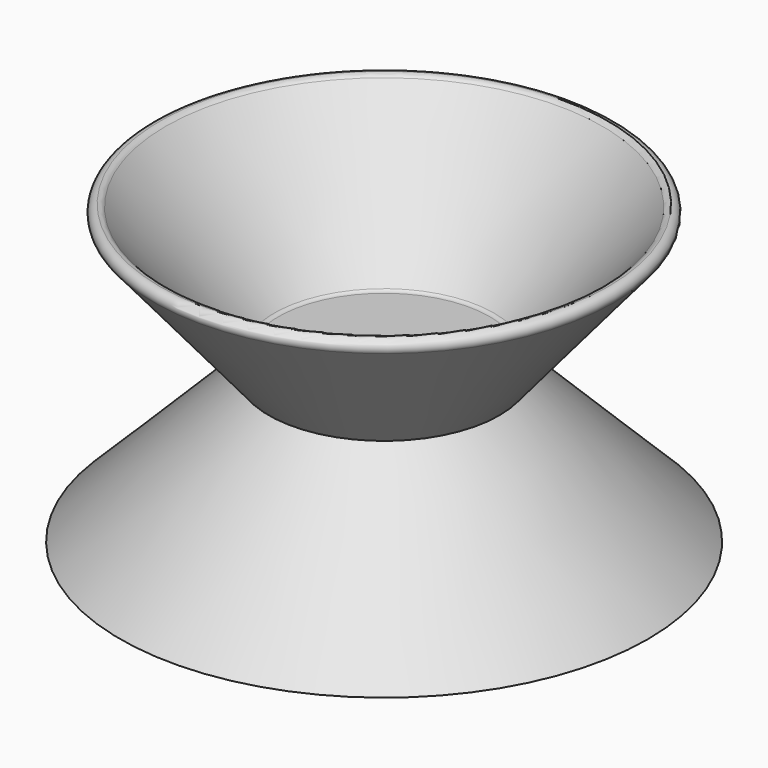
from build123d import *

# Parameters (mm, degrees)
F0_R      = 49.2737208463
F1_DEPTH  = 63.5
F1_TAPER  = -40
F2_T      = -6.35
F3_R      = 3.17499
F1_FACE_R = 49.2737208463
F4_DEPTH  = 63.5
F4_TAPER  = -45
F5_T      = -6.35
F6_R      = 2.286


# Not quite as in the source:
# - a fillet or chamfer that OpenCascade refuses, or shapes differently, is made with other operations: its cross-section is extruded or revolved along the edge and cut away or added
# - a fillet or chamfer is up to 0.001 mm smaller than in the source, because OpenCascade refuses the exact size


with BuildPart() as f1:
    # F0 (on Top) → F1 (new body)
    with BuildSketch(Plane.XY):
        Circle(F0_R)
    extrude(amount=F1_DEPTH, taper=F1_TAPER)

    # F2
    f2_openings = [f1.faces().sort_by_distance(p)[0] for p in [
        (0, 0, 63.5),
    ]]
    offset(amount=F2_T, openings=f2_openings, kind=Kind.INTERSECTION)

    # F3 (radius 3.175 in the source; OpenCascade refuses exactly that, so slightly less here)
    f3_edges = [f1.edges().sort_by_distance(p)[0] for p in [
        (-102.556547, 0, 63.5),
        (-94.267211, 0, 63.5),
    ]]
    fillet(f3_edges, radius=F3_R)

    # F1_face (on face) → F4 (join)
    with BuildSketch(Plane(origin=(0, 0, 0), x_dir=(1, 0, 0), z_dir=(0, 0, -1))):
        Circle(F1_FACE_R)
    extrude(amount=F4_DEPTH, taper=F4_TAPER)

    # F5
    f5_openings = [f1.faces().sort_by_distance(p)[0] for p in [
        (0, 0, -63.5),
    ]]
    offset(amount=F5_T, openings=f5_openings, kind=Kind.INTERSECTION)

    # F6
    f6_edges = [f1.edges().sort_by_distance(p)[0] for p in [
        (-46.312667, 0, 6.35),
    ]]
    fillet(f6_edges, radius=F6_R)

    # F7: fillet of radius 2.286 on 1 edges, made by hand

    # F7_s1 → F7_t2 (revolve, cut)
    with BuildSketch(Plane.XZ):
        with BuildLine():
            ThreePointArc((41.6376699139, -1.3442051886), (41.1980722658, -0.7269988473), (40.984384559, 0))
            Line((40.984384559, 0), (40.6691484685, -0.3756837433))
            Line((40.6691484685, -0.3756837433), (41.6376699139, -1.3442051886))
        make_face()
    revolve(axis=Axis((0, 0, -0.3756837433), (0, 0, 1)), mode=Mode.SUBTRACT)


solid = f1.part
